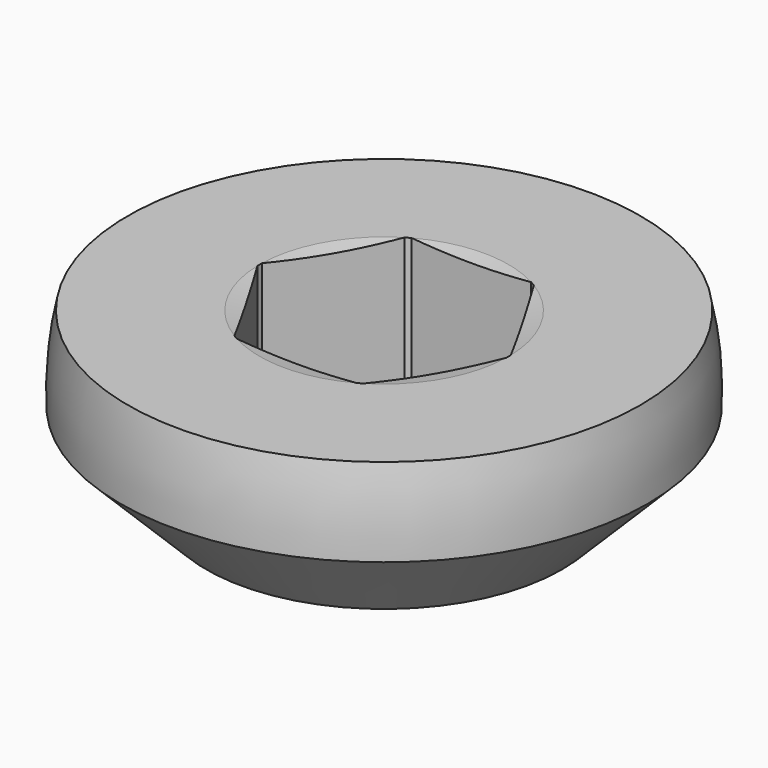
from build123d import *

# Parameters (mm, degrees)
F2_R     = 6.7823339415
F3_DEPTH = 8.07
F4_R     = 5.9
F5_DEPTH = 1
F5_TAPER = 80


# Not quite as in the source:
# - an extrude ends at something that could not be found from the text; its depth is read off the source's solid


with BuildPart() as f1:
    # F0 (on Front) → F1 (revolve)
    with BuildSketch(Plane.XZ):
        with BuildLine():
            Line((12.1487583965, 8.07), (5.9, 8.07))
            Line((5.9, 8.07), (5.9, 1.82))
            Line((5.9, 1.82), (2.7476675302, 0))
            Line((2.7476675302, 0), (8.43, 0))
            Line((8.43, 0), (12.5, 4.07))
            ThreePointArc((12.5, 4.07), (12.4588304791, 6.0818062209), (12.1487583965, 8.07))
        make_face()
    revolve(axis=Axis((0, 0, -0.4323393759), (0, 0, 1)))

    # F2 (on face) → F3 (join, through all)
    with BuildSketch(Plane.XY.offset(8.07)):
        Circle(F2_R)
        Polygon((-5.9755752861, 0), (-2.9877876431, 5.175), (2.9877876431, 5.175), (5.9755752861, 0), (2.9877876431, -5.175), (-2.9877876431, -5.175), align=None, mode=Mode.SUBTRACT)
    extrude(amount=-F3_DEPTH)

    # F4 (on face) → F5 (cut)
    with BuildSketch(Plane.XY.offset(8.07)):
        Circle(F4_R)
    extrude(amount=-F5_DEPTH, taper=F5_TAPER, mode=Mode.SUBTRACT)


solid = f1.part
